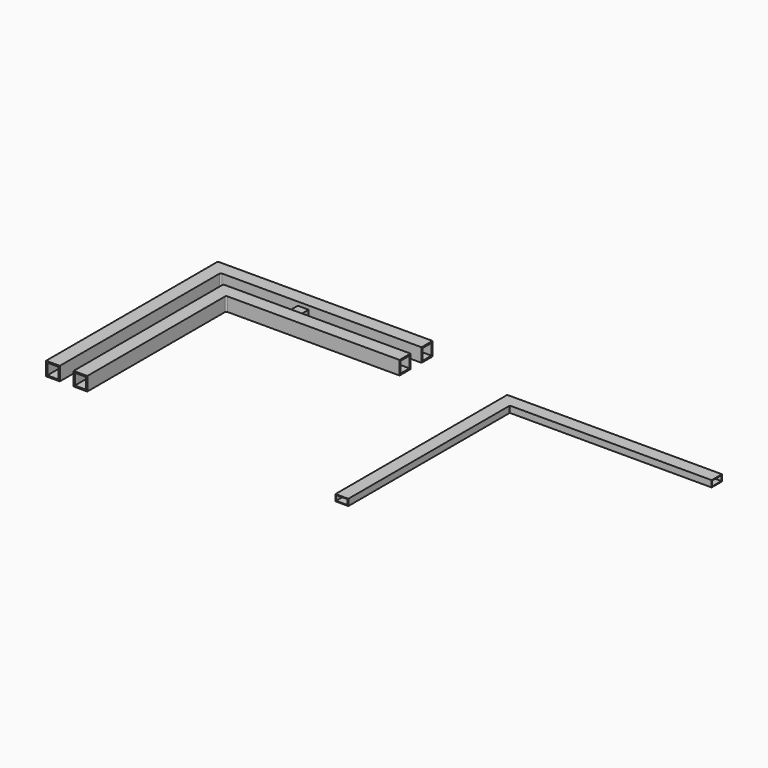
from build123d import *

# Parameters (mm, degrees)
F1_DEPTH      = 16
F1_DEPTH_BACK = 16
F2_R          = 3
F2_2_R        = 3
F3_T          = 3
F3_2_T        = 3
F4_W          = 25
F4_H          = 32
F5_DEPTH      = 7.5
F5_DEPTH_BACK = 7.5
F7_DEPTH      = 7.5
F7_DEPTH_BACK = 7.5
F8_R          = 1.5
F9_T          = 1.5


# Not quite as in the source:
# - a shell that OpenCascade refuses in one call is made with other operations: the cavity is built on its own and cut out


with BuildPart() as f1:
    # F0 (on Top) → F1 (new body, two sides)
    with BuildSketch(Plane.XY) as f1_sk:
        Polygon((500, -64), (64, -64), (64, -500), (96, -500), (96, -96), (500, -96), align=None)
    extrude(amount=F1_DEPTH)
    extrude(f1_sk.sketch, amount=-F1_DEPTH_BACK)

    # F2
    f2_edges = [f1.edges().sort_by_distance(p)[0] for p in [
        (64, -64, 0),
        (96, -96, 0),
    ]]
    fillet(f2_edges, radius=F2_R)

    # F3#2: shell of thickness 3, made by hand


with BuildPart() as f1b:
    # F0 (on Top) → F1, piece 2 (new body, two sides)
    with BuildSketch(Plane.XY) as f1_2_sk:
        Polygon((500, 0), (0, 0), (0, -500), (32, -500), (32, -32), (500, -32), align=None)
    extrude(amount=F1_DEPTH)
    extrude(f1_2_sk.sketch, amount=-F1_DEPTH_BACK)

    # F2#2
    f2_2_edges = [f1b.edges().sort_by_distance(p)[0] for p in [
        (0, 0, 0),
        (32, -32, 0),
    ]]
    fillet(f2_2_edges, radius=F2_2_R)

    # F3: shell of thickness 3, made by hand


with BuildPart() as f3_core1:
    # F3_t2: copy of F1b
    add(f1b.part)

    # the walls: a layer under each face that stays
    f3_faces = [f3_core1.faces().sort_by_distance(p)[0] for p in [
        (251.5, 0, 0),
        (16.6666666667, -483.3333333333, 16),
        (16.6666666667, -483.3333333333, -16),
        (0, -251.5, 0),
        (267.5, -32, 0),
        (32.8786796564, -32.8786796564, 0),
        (32, -267.5, 0),
    ]]
    thicken(f3_faces, amount=-F3_T, mode=Mode.SUBTRACT)


with BuildPart() as f1b_1:
    add(f1b.part)

    # what is left inside the walls is the cavity
    f3_cavity = [f3_core1.part.solids().sort_by_distance(p)[0] for p in [
        (18.53125, -205.481481, -12.97),
    ]]
    add(f3_cavity, mode=Mode.SUBTRACT)


with BuildPart() as f3_2_core1:
    # F3_2_t2: copy of F1
    add(f1.part)

    # the walls: a layer under each face that stays
    f3_2_faces = [f3_2_core1.faces().sort_by_distance(p)[0] for p in [
        (283.5, -64, 0),
        (95.1428571429, -468.8571428571, 16),
        (95.1428571429, -468.8571428571, -16),
        (64, -283.5, 0),
        (299.5, -96, 0),
        (96.8786796564, -96.8786796564, 0),
        (96, -299.5, 0),
    ]]
    thicken(f3_2_faces, amount=-F3_2_T, mode=Mode.SUBTRACT)


with BuildPart() as f1_1:
    add(f1.part)

    # what is left inside the walls is the cavity
    f3_2_cavity = [f3_2_core1.part.solids().sort_by_distance(p)[0] for p in [
        (80.53125, -243.407407, -12.97),
    ]]
    add(f3_2_cavity, mode=Mode.SUBTRACT)


with BuildPart() as f5:
    # F4 (on Top) → F5 (new body, two sides)
    with BuildSketch(Plane.XY) as f5_sk:
        with Locations((224.534201622, -48)):
            Rectangle(F4_W, F4_H)
    extrude(amount=F5_DEPTH)
    extrude(f5_sk.sketch, amount=-F5_DEPTH_BACK)


with BuildPart() as f7:
    # F6 (on Top) → F7 (new body, two sides)
    with BuildSketch(Plane.XY) as f7_sk:
        Polygon((1228.6461293697, -68.4013846497), (728.6461293697, -68.4013846497), (728.6461293697, -568.4013846497), (758.6461293697, -568.4013846497), (758.6461293697, -98.4013846497), (1228.6461293697, -98.4013846497), align=None)
    extrude(amount=F7_DEPTH)
    extrude(f7_sk.sketch, amount=-F7_DEPTH_BACK)

    # F8
    f8_edges = [f7.edges().sort_by_distance(p)[0] for p in [
        (728.646129, -68.401385, 0),
        (758.646129, -98.401385, 0),
    ]]
    fillet(f8_edges, radius=F8_R)

    # F9: shell of thickness 1.5, made by hand


with BuildPart() as f9_core1:
    # F9_t2: copy of F7
    add(f7.part)

    # the walls: a layer under each face that stays
    f9_faces = [f9_core1.faces().sort_by_distance(p)[0] for p in [
        (979.3961293697, -68.4013846497, 0),
        (745.3127960364, -551.7347179831, 7.5),
        (745.3127960364, -551.7347179831, -7.5),
        (728.6461293697, -319.1513846497, 0),
        (994.3961293697, -98.4013846497, 0),
        (759.085469198, -98.840724478, 0),
        (758.6461293697, -334.1513846497, 0),
    ]]
    thicken(f9_faces, amount=-F9_T, mode=Mode.SUBTRACT)


with BuildPart() as f7_1:
    add(f7.part)

    # what is left inside the walls is the cavity
    f9_cavity = [f9_core1.part.solids().sort_by_distance(p)[0] for p in [
        (745.724254, -272.993977, -5.985),
    ]]
    add(f9_cavity, mode=Mode.SUBTRACT)


solid = Compound([f1b_1.part, f1_1.part, f5.part, f7_1.part])
